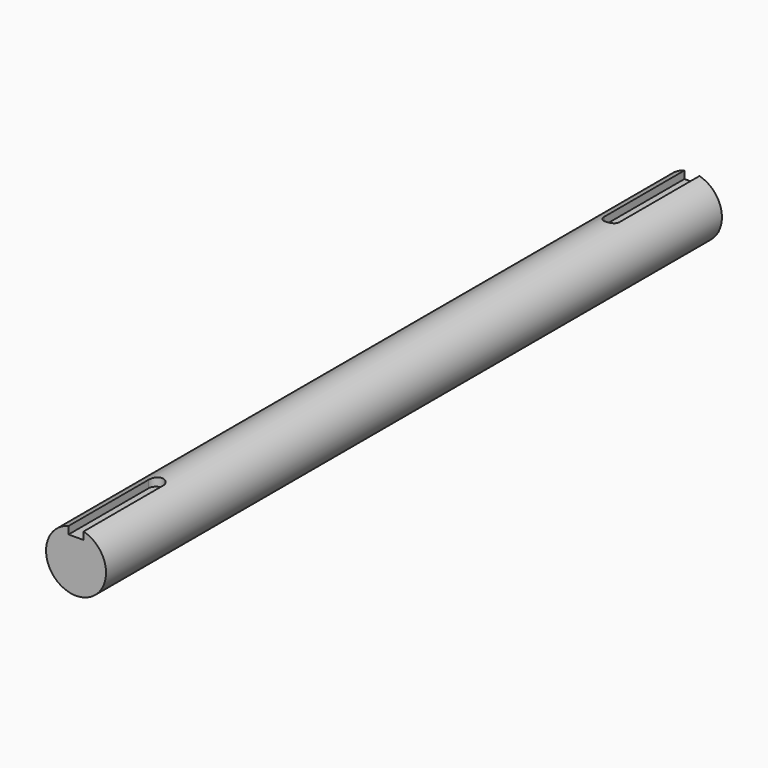
from build123d import *

# Parameters (mm, degrees)
F0_R     = 38.1
F1_DEPTH = 488.95
F4_DEPTH = 10.7442


# Not quite as in the source:
# - a pattern or mirror of a feature is missing from the dataset's text; its kind, count and spacing are read off the source's solid


with BuildPart() as f1:
    # F0 (on Front) → F1 (new body, symmetric)
    with BuildSketch(Plane.XZ):
        Circle(F0_R)
    extrude(amount=F1_DEPTH, both=True)

    # F3 (on offset) → F4 (cut)
    with BuildSketch(Plane.XY.offset(38.1)):
        with BuildLine():
            Line((-9.525, -361.95), (-9.525, -574.1807818413))
            Line((-9.525, -574.1807818413), (9.525, -574.1807818413))
            Line((9.525, -574.1807818413), (9.525, -361.95))
            ThreePointArc((9.525, -361.95), (0, -352.425), (-9.525, -361.95))
        make_face()
    f4 = extrude(amount=-F4_DEPTH, mode=Mode.SUBTRACT)

    # F4_copies: F4 across plane
    add(f4.mirror(Plane.ZX), mode=Mode.SUBTRACT)


solid = f1.part
